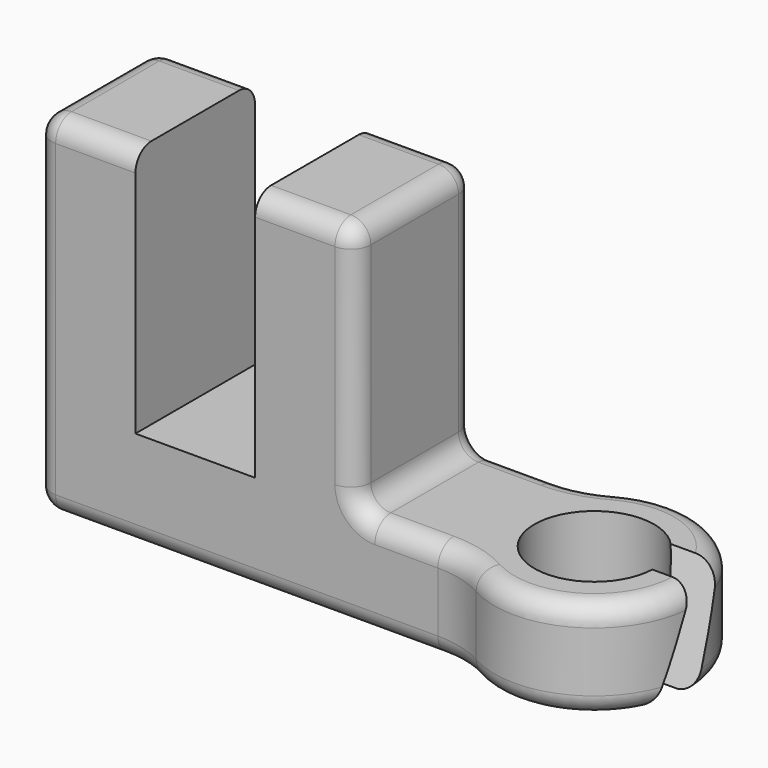
from build123d import *

# Parameters (mm, degrees)
F0_R     = 3.81
F1_DEPTH = 6.35
F2_W     = 6.35
F2_H     = 9.5123
F3_DEPTH = 15.875
F4_R     = 1.27
F6_DEPTH = 6.351


with BuildPart() as f1:
    # F0 (on Top) → F1 (new body)
    with BuildSketch(Plane.XY):
        with BuildLine():
            ThreePointArc((-6.1483610621, -4.7625), (-4.5608610621, -4.9641389379), (-3.0741805311, -5.55625))
            ThreePointArc((-3.0741805311, -5.55625), (6.3499966259, 0.0065460587), (-3.0856295938, 5.5499))
            ThreePointArc((-3.0856295938, 5.5499), (-4.577421837, 4.9530787195), (-6.1712591876, 4.7498))
            Line((-6.1712591876, 4.7498), (-31.75, 4.7498))
            Line((-31.75, 4.7498), (-31.75, -4.7625))
            Line((-31.75, -4.7625), (-6.1483610621, -4.7625))
        make_face()
        Circle(F0_R, mode=Mode.SUBTRACT)
    extrude(amount=F1_DEPTH)

    # F2 (on face) → F3 (join)
    with BuildSketch(Plane.XY.offset(6.35)):
        with Locations((-28.575, -0.00635)):
            Rectangle(F2_W, F2_H)
        with Locations((-14.605, -0.00635)):
            Rectangle(F2_W, F2_H)
    extrude(amount=F3_DEPTH)

    # F4
    f4_edges = [f1.edges().sort_by_distance(p)[0] for p in [
        (-18.949181, -4.7625, 0),
        (-8.789181, -4.7625, 6.35),
        (-11.43, -0.00635, 6.35),
        (-11.43, -0.00635, 22.225),
        (-31.75, -4.7625, 11.1125),
        (-31.75, -0.00635, 0),
        (-31.75, 4.7498, 11.1125),
        (-28.575, -4.7625, 22.225),
        (-31.75, -0.00635, 22.225),
        (-28.575, 4.7498, 22.225),
        (-14.605, -4.7625, 22.225),
        (-14.605, 4.7498, 22.225),
        (-4.560861, -4.964139, 0),
        (-4.560861, -4.964139, 6.35),
        (-4.577422, 4.953079, 6.35),
        (-4.577422, 4.953079, 0),
        (-11.43, 4.7498, 14.2875),
        (-18.96063, 4.7498, 0),
        (-11.43, -4.7625, 14.2875),
    ]]
    fillet(f4_edges, radius=F4_R)

    # F5 (on Right) → F6 (cut, through all)
    with BuildSketch(Plane.YZ):
        Polygon((-4.3603489199, -4.6240965693), (-1.9896510801, -5.5359034307), (4.3603489199, 10.9740965693), (1.9896510801, 11.8859034307), align=None)
    extrude(amount=F6_DEPTH, mode=Mode.SUBTRACT)


solid = f1.part
